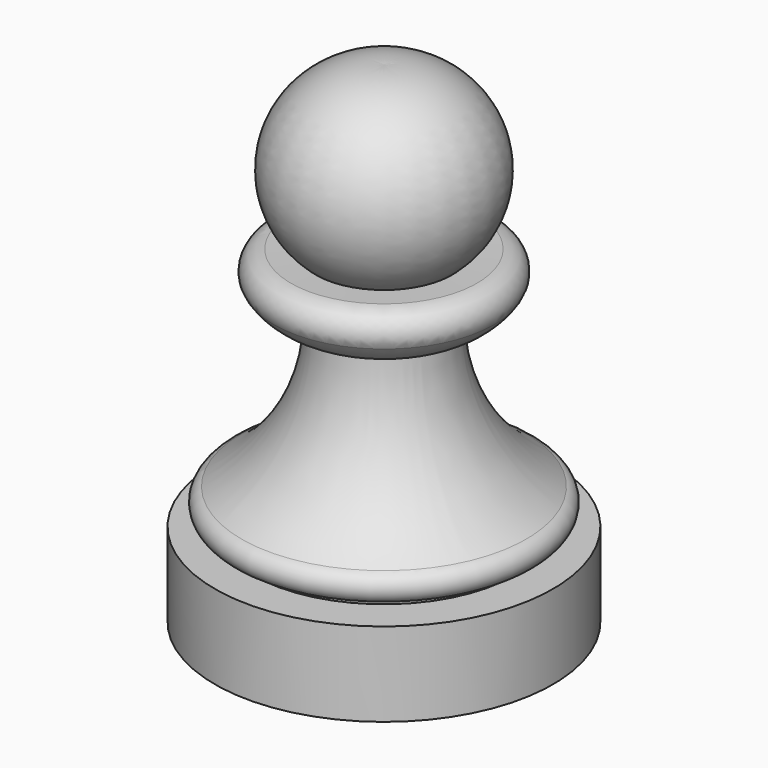
from build123d import *

# Parameters (mm, degrees)
F0_W = 13.7083213776
F0_H = 6.8093617447
F9_R = 1.6073014862


# Not quite as in the source:
# - a fillet or chamfer that OpenCascade refuses, or shapes differently, is made with other operations: its cross-section is extruded or revolved along the edge and cut away or added


with BuildPart() as f1:
    # F0 (on Front) → F1 (revolve)
    with BuildSketch(Plane.XZ):
        with Locations((-6.8541606888, 3.4046808723)):
            Rectangle(F0_W, F0_H)
    revolve(axis=Axis((0, 0, 3.4046808723), (0, 0, -1)))

    # F2 (on Front) → F3 (revolve)
    with BuildSketch(Plane.XZ):
        with BuildLine():
            ThreePointArc((-5.1070209593, 21.6824412346), (-6.8126416021, 14.8628068286), (-11.5579944104, 9.676461108))
            ThreePointArc((-11.5579944104, 9.676461108), (-12.2502768318, 8.1261884439), (-10.6620267034, 7.5261369348))
            Line((-10.6620267034, 7.5261369348), (-10.6620267034, 6.6301682964))
            Line((-10.6620267034, 6.6301682964), (0, 6.6301682964))
            Line((0, 6.6301682964), (0, 21.6824412346))
            Line((0, 21.6824412346), (-5.1070209593, 21.6824412346))
        make_face()
    revolve(axis=Axis((0, 0, 14.1563047655), (0, 0, -1)))


with BuildPart() as f5:
    # F4 (on Front) → F5 (revolve)
    with BuildSketch(Plane.XZ):
        Polygon((-9.781897068, 21.8616351485), (-4.748633597, 21.8616351485), (0, 21.8616351485), (0, 26.5206731856), (-4.2110513896, 26.5206731856), (-9.781897068, 26.7053246498), align=None)
    revolve(axis=Axis((0, 0, 24.1911541671), (0, 0, -1)))

    # F6 (on Front) → F7 (revolve)
    with BuildSketch(Plane.XZ):
        with BuildLine():
            Line((0, 26.2412168086), (0, 39.7947132587))
            ThreePointArc((0, 39.7947132587), (-7.6776526733, 34.9494378225), (-5.1105665043, 26.2412168086))
            Line((-5.1105665043, 26.2412168086), (0, 26.2412168086))
        make_face()
    revolve(axis=Axis((0, 0, 33.0179650337), (0, 0, 1)))

    # F8: fillet of radius 5.08 on 1 edges, made by hand

    # F8_s1 → F8_t2 (revolve, cut)
    with BuildSketch(Plane.XZ):
        with BuildLine():
            ThreePointArc((-9.781897068, 26.7053246498), (-8.2149555389, 23.2669339815), (-4.7073963686, 21.8616351485))
            Line((-4.7073963686, 21.8616351485), (-9.781897068, 21.8616351485))
            Line((-9.781897068, 21.8616351485), (-9.781897068, 26.7053246498))
        make_face()
    revolve(axis=Axis((0, 0, 21.8616351485), (0, 0, -1)), mode=Mode.SUBTRACT)

    # F9
    f9_edges = [f5.edges().sort_by_distance(p)[0] for p in [
        (9.781897, 0, 26.705325),
    ]]
    fillet(f9_edges, radius=F9_R)


solid = Compound([f1.part, f5.part])
